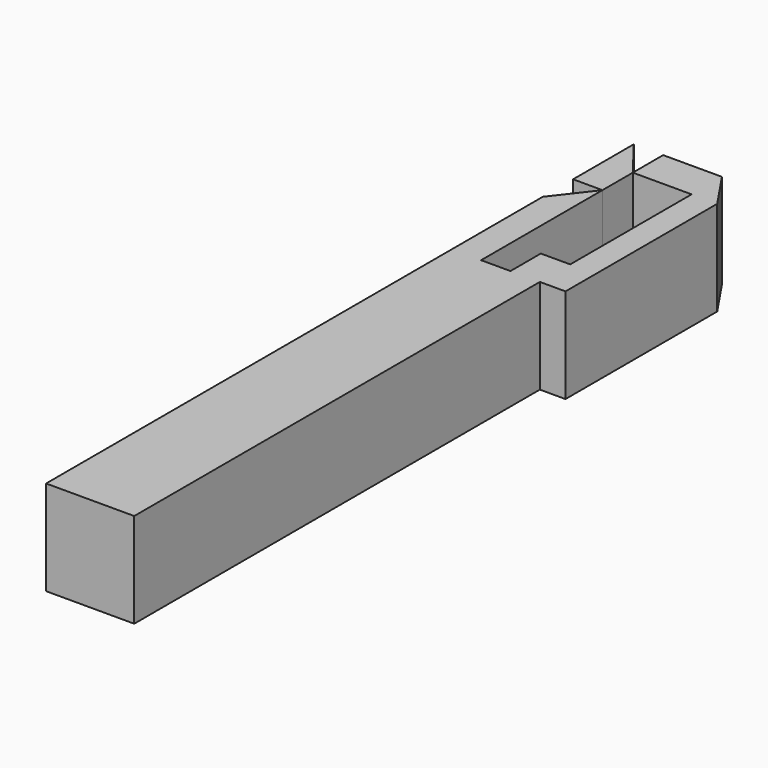
from build123d import *

# Parameters (mm, degrees)
F0_W     = 7.7470013483
F0_H     = 133.6750337083
F0_H_2   = 10
F0_W_2   = 6.758995955
F1_DEPTH = 25


with BuildPart() as f1:
    # F0 (on Top) → F1 (new body)
    with BuildSketch(Plane.XY):
        with Locations((0, -30)):
            Rectangle(F0_W, F0_H)
        with Locations((-7.7470013483, -30)):
            Rectangle(F0_W, F0_H)
        with Locations((7.7470013483, -30)):
            Rectangle(F0_W, F0_H)
        with Locations((-7.7470013483, 41.8375168541)):
            Rectangle(F0_W, F0_H_2)
        Polygon((3.8735006742, 46.8375168541), (3.8735006742, 36.8375168541), (11.6205020225, 36.8375168541), (11.6205020225, 46.8375168541), (8.7326292689, 46.8375168541), align=None)
        Polygon((-11.6205020225, 56.8375168541), (-3.8735006742, 46.8375168541), (-3.8735006742, 56.8375168541), align=None)
        Polygon((-11.6205020225, 46.8375168541), (-3.8735006742, 46.8375168541), (-11.6205020225, 56.8375168541), align=None)
        with Locations((15, 41.8375168541)):
            Rectangle(F0_W_2, F0_H_2)
        with Locations((-7.7470013483, 61.8375168541)):
            Rectangle(F0_W, F0_H_2)
        with Locations((15, 51.8375168541)):
            Rectangle(F0_W_2, F0_H_2)
        Polygon((-11.6205020225, 66.8375168541), (-3.8735006742, 66.8375168541), (-3.8735006742, 76.8375168541), align=None)
        with Locations((15, 61.8375168541)):
            Rectangle(F0_W_2, F0_H_2)
        Polygon((18.3794979775, 76.8375168541), (11.6205020225, 66.8375168541), (18.3794979775, 66.8375168541), align=None)
        Polygon((11.6205020225, 76.8375168541), (11.6205020225, 66.8375168541), (18.3794979775, 76.8375168541), align=None)
        with Locations((0, 91.8375168541)):
            Rectangle(F0_W, F0_H_2)
        with Locations((7.7470013483, 91.8375168541)):
            Rectangle(F0_W, F0_H_2)
        with Locations((15, 81.8375168541)):
            Rectangle(F0_W_2, F0_H_2)
        Polygon((11.6205020225, 96.8375168541), (11.6205020225, 86.8375168541), (18.3794979775, 86.8375168541), align=None)
    extrude(amount=F1_DEPTH)


with BuildPart() as f1b:
    # F0 (on Top) → F1, piece 2 (new body)
    with BuildSketch(Plane.XY):
        with Locations((-7.7470013483, 81.8375168541)):
            Rectangle(F0_W, F0_H_2)
        Polygon((-11.6205020225, 86.8375168541), (-3.8735006742, 86.8375168541), (-11.6205020225, 96.8375168541), align=None)
    extrude(amount=F1_DEPTH)


solid = Compound([f1.part, f1b.part])
